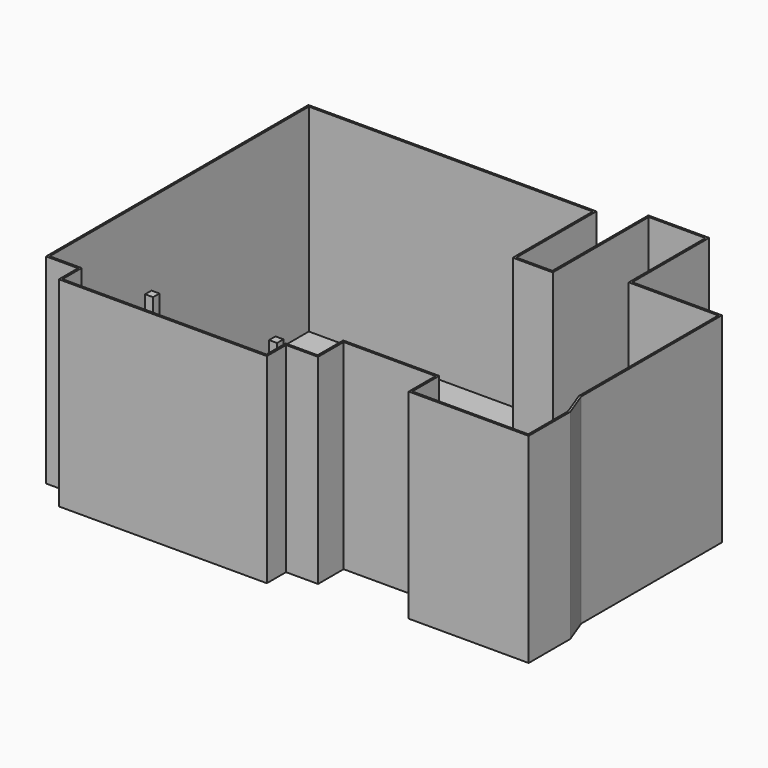
from build123d import *

# Parameters (mm, degrees)
F1_DEPTH = 250
F2_T     = -2.5
F3_W     = 200
F3_H     = 1.5
F4_DEPTH = 60
F6_DEPTH = 200
F8_DEPTH = 200
F7_W     = 145
F7_H     = 4.445284605
F9_DEPTH = 130


with BuildPart() as f1:
    # F0 (on Top) → F1 (new body)
    with BuildSketch(Plane.XY):
        Polygon((104.6832542723, 230.6472660226), (-255.3167457277, 230.6472660226), (-255.3167457277, -179.3527339774), (-215.3167457277, -179.3527339774), (-215.3167457277, -209.3527339774), (44.6832542723, -209.3527339774), (44.6832542723, -179.3527339774), (84.6832542723, -179.3527339774), (84.6832542723, -139.3527339774), (199.6832542723, -139.3527339774), (199.6832542723, -181.3527339774), (349.6832542723, -181.3527339774), (349.6832542723, -116.3527339774), (337.6832542723, -84.3527339774), (337.6832542723, 135.6472660226), (225.6832542723, 135.6472660226), (225.6832542723, 255.6472660226), (149.6832542723, 255.6472660226), (149.6832542723, 105.6472660226), (104.6832542723, 105.6472660226), align=None)
    extrude(amount=F1_DEPTH)

    # F2
    f2_openings = [f1.faces().sort_by_distance(p)[0] for p in [
        (24.63536, 12.151901, 250),
    ]]
    offset(amount=F2_T, openings=f2_openings, kind=Kind.INTERSECTION)

    # F3 (on face) → F4 (join)
    with BuildSketch(Plane.XY.offset(2.5)):
        with Locations((-112.8167457277, -175.5136670351)):
            Rectangle(F3_W, F3_H)
    extrude(amount=F4_DEPTH)

    # F5 (on face) → F6 (join)
    with BuildSketch(Plane.YZ.offset(-12.8167457277)):
        Polygon((-127.7790359959, 76.1753777748), (-174.7636670351, 59.0743706086), (-174.7636670351, 2.5), (-127.7790359959, 2.5), align=None)
    extrude(amount=-F6_DEPTH)


with BuildPart() as f8:
    # F7 (on face) → F8 (new body)
    with BuildSketch(Plane.XY.offset(2.5)):
        Polygon((-176.8384825487, -100.2069843521), (-186.8384825487, -100.2069843521), (-186.8384825487, -110.2069843521), (-176.8384825487, -110.2069843521), (-176.8384825487, -107.1964427829), (-176.8384825487, -102.7511581779), align=None)
    extrude(amount=F8_DEPTH)


with BuildPart() as f8b:
    # F7 (on face) → F8, piece 2 (new body)
    with BuildSketch(Plane.XY.offset(2.5)):
        Polygon((-31.8384825487, -100.2069843521), (-31.8384825487, -102.7511581779), (-31.8384825487, -107.1964427829), (-31.8384825487, -110.2069843521), (-21.8384855244, -110.2069843521), (-21.8384855244, -100.2069843521), align=None)
    extrude(amount=F8_DEPTH)


with BuildPart() as f9:
    # F7 (on face) → F9 (new body)
    with BuildSketch(Plane.XY.offset(2.5)):
        with Locations((-104.3384825487, -104.9738004804)):
            Rectangle(F7_W, F7_H)
    extrude(amount=F9_DEPTH)


solid = Compound([f1.part, f8.part, f8b.part, f9.part])
